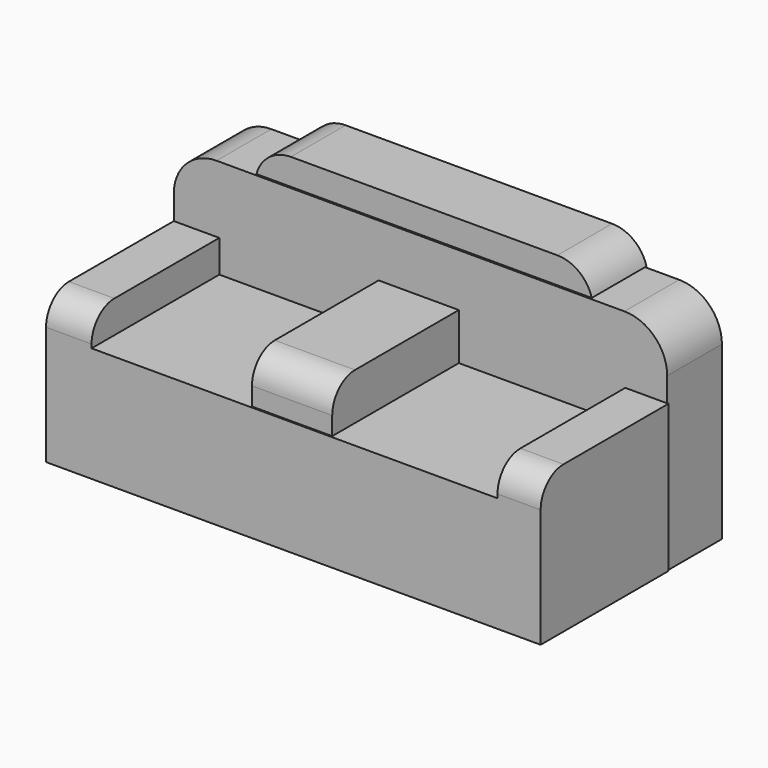
from build123d import *

# Parameters (mm, degrees)
F0_W         = 72.3290368915
F0_H         = 20.4825587571
F1_DEPTH     = 28.448
F2_W         = 87.9043228924
F2_H         = 38.1914395839
F3_DEPTH     = 12.192
F4_W         = 14.2951197922
F4_H         = 8.3210412413
F5_DEPTH     = 28.194
F6_R         = 5.08
F7_R         = 5.08
F8_R         = 7.62
F9_R         = 7.62
F10_W        = 59.7411263734
F10_H        = 4.6939216554
F11_DEPTH    = 12.192
F12_T1_DEPTH = 42.8432253085
F13_T1_DEPTH = 42.8432253085


# Not quite as in the source:
# - a fillet or chamfer that OpenCascade refuses, or shapes differently, is made with other operations: its cross-section is extruded or revolved along the edge and cut away or added


with BuildPart() as f1:
    # F0 (on Front) → F1 (new body)
    with BuildSketch(Plane.XZ):
        Polygon((-24.7497595847, -56.5403997898), (-24.7497595847, -36.0578410327), (-24.7497595847, -30.2971210331), (-32.857440412, -30.2971210331), (-32.857440412, -56.5403997898), align=None)
        Polygon((47.5792773068, -30.2971210331), (47.5792773068, -36.0578410327), (47.5792773068, -56.5403997898), (55.2602447569, -56.5403997898), (55.2602447569, -30.2971210331), align=None)
        with Locations((11.4147588611, -46.2991204113)):
            Rectangle(F0_W, F0_H)
    extrude(amount=F1_DEPTH)

    # F2 (on Front) → F3 (join)
    with BuildSketch(Plane.XZ):
        with Locations((11.0947210342, -37.4446799979)):
            Rectangle(F2_W, F2_H)
    extrude(amount=-F3_DEPTH)

    # F4 (on Front) → F5 (join)
    with BuildSketch(Plane.XZ):
        with Locations((10.774679482, -31.8973204121)):
            Rectangle(F4_W, F4_H)
    extrude(amount=F5_DEPTH)

    # F6
    f6_edges = [f1.edges().sort_by_distance(p)[0] for p in [
        (10.774679, -28.194, -27.7368),
    ]]
    fillet(f6_edges, radius=F6_R)

    # F7
    f7_edges = [f1.edges().sort_by_distance(p)[0] for p in [
        (51.419761, -28.448, -30.297121),
        (-28.8036, -28.448, -30.297121),
    ]]
    fillet(f7_edges, radius=F7_R)

    # F8
    f8_edges = [f1.edges().sort_by_distance(p)[0] for p in [
        (55.046882, 6.096, -18.34896),
    ]]
    fillet(f8_edges, radius=F8_R)

    # F9
    f9_edges = [f1.edges().sort_by_distance(p)[0] for p in [
        (-32.85744, 6.096, -18.34896),
    ]]
    fillet(f9_edges, radius=F9_R)


with BuildPart() as f11:
    # F10 (on Front) → F11 (new body)
    with BuildSketch(Plane.XZ):
        with Locations((11.7347566411, -15.7886408269)):
            Rectangle(F10_W, F10_H)
    extrude(amount=-F11_DEPTH)

    # F12: fillet of radius 6.35 on 1 edges, made by hand

    # F12_s2 → F12_t1 (cut)
    with BuildSketch(Plane.XZ.offset(-27.5176126543)):
        with BuildLine():
            ThreePointArc((41.6053198278, -18.1356016546), (39.3355412218, -14.7499244772), (35.4750747661, -13.4416799992))
            Line((35.4750747661, -13.4416799992), (41.6053198278, -13.4416799992))
            Line((41.6053198278, -13.4416799992), (41.6053198278, -18.1356016546))
        make_face()
    extrude(amount=F12_T1_DEPTH, mode=Mode.SUBTRACT)

    # F13: fillet of radius 6.35 on 1 edges, made by hand

    # F13_s2 → F13_t1 (cut)
    with BuildSketch(Plane.XZ.offset(-27.5176126543)):
        with BuildLine():
            ThreePointArc((-18.1358065456, -18.1356016546), (-15.8660279397, -14.7499244772), (-12.0055614839, -13.4416799992))
            Line((-12.0055614839, -13.4416799992), (-18.1358065456, -13.4416799992))
            Line((-18.1358065456, -13.4416799992), (-18.1358065456, -18.1356016546))
        make_face()
    extrude(amount=F13_T1_DEPTH, mode=Mode.SUBTRACT)


solid = Compound([f1.part, f11.part])
